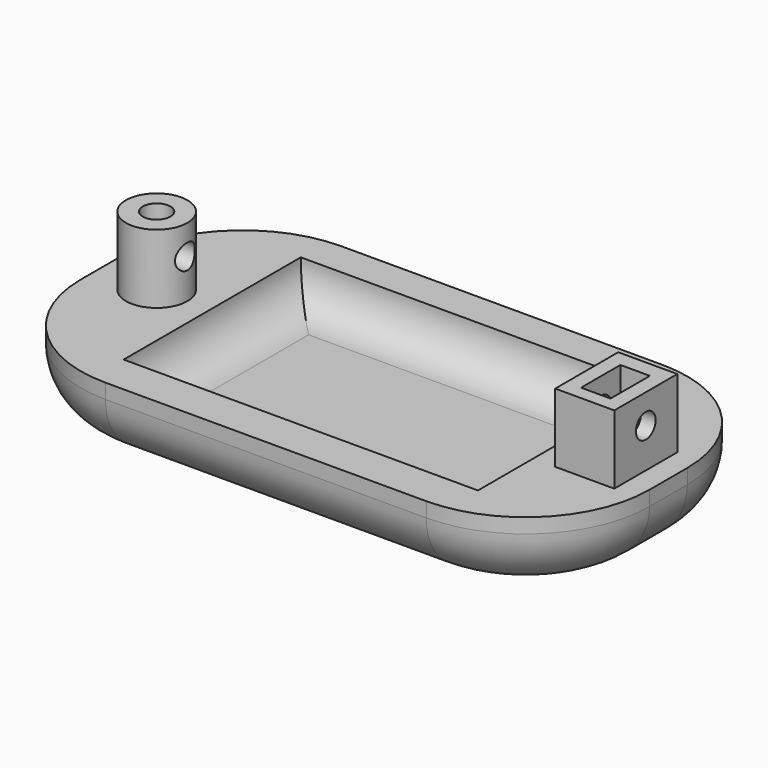
from build123d import *

# Parameters (mm, degrees)
F0_W      = 73.406
F0_H      = 38.1
F1_DEPTH  = 9.525
F2_R      = 16.002
F3_R      = 3.96875
F3_W      = 7.62
F3_H      = 10.16
F4_DEPTH  = 8.89
F5_R      = 1.5875
F6_DEPTH  = 68.58
F7_R      = 1.778
F7_W      = 3.81
F7_H      = 6.35
F8_DEPTH  = 12.7
F9_R      = 7.62
F10_W     = 45.72
F10_H     = 28.575
F11_DEPTH = 5.08
F12_R     = 5.07999


# Not quite as in the source:
# - a fillet or chamfer is up to 0.001 mm smaller than in the source, because OpenCascade refuses the exact size


with BuildPart() as f1:
    # F0 (on Top) → F1 (new body)
    with BuildSketch(Plane.XY):
        with Locations((36.703, 19.05)):
            Rectangle(F0_W, F0_H)
    extrude(amount=F1_DEPTH)

    # F2
    f2_edges = [f1.edges().sort_by_distance(p)[0] for p in [
        (0, 38.1, 4.7625),
        (0, 0, 4.7625),
        (73.406, 38.1, 4.7625),
        (73.406, 0, 4.7625),
    ]]
    fillet(f2_edges, radius=F2_R)

    # F3 (on face) → F4 (join)
    with BuildSketch(Plane.XY.offset(9.525)):
        with Locations((7.366, 19.05)):
            Circle(F3_R)
        with Locations((66.675, 19.05)):
            Rectangle(F3_W, F3_H)
    extrude(amount=F4_DEPTH)

    # F5 (on face) → F6 (cut)
    with BuildSketch(Plane.YZ.offset(70.485)):
        with Locations((19.05, 14.605)):
            Circle(F5_R)
    extrude(amount=-F6_DEPTH, mode=Mode.SUBTRACT)

    # F7 (on face) → F8 (cut)
    with BuildSketch(Plane.XY.offset(18.415)):
        with Locations((7.366, 19.05)):
            Circle(F7_R)
        with Locations((66.675, 18.923)):
            Rectangle(F7_W, F7_H)
    extrude(amount=-F8_DEPTH, mode=Mode.SUBTRACT)

    # F9
    f9_edges = [f1.edges().sort_by_distance(p)[0] for p in [
        (36.703, 0, 0),
    ]]
    fillet(f9_edges, radius=F9_R)

    # F10 (on face) → F11 (cut)
    with BuildSketch(Plane.XY.offset(9.525)):
        with Locations((37.1440443242, 19.3675)):
            Rectangle(F10_W, F10_H)
    extrude(amount=-F11_DEPTH, mode=Mode.SUBTRACT)

    # F12 (radius 5.08 in the source; OpenCascade refuses exactly that, so slightly less here)
    f12_edges = [f1.edges().sort_by_distance(p)[0] for p in [
        (60.004044, 19.3675, 4.445),
        (37.144044, 33.655, 4.445),
        (14.284044, 19.3675, 4.445),
        (37.144044, 5.08, 4.445),
    ]]
    fillet(f12_edges, radius=F12_R)


solid = f1.part
